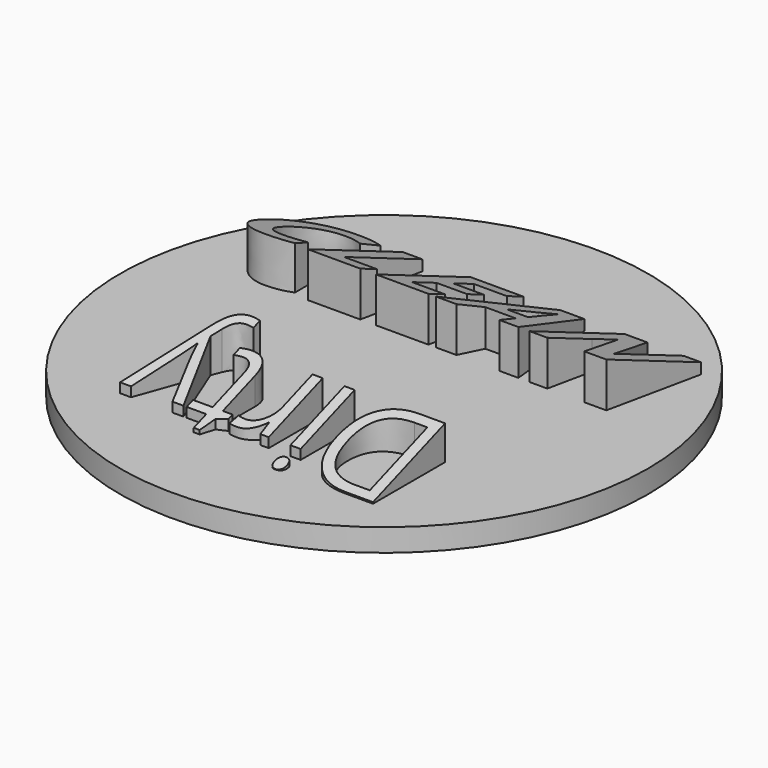
from build123d import *

# Parameters (mm, degrees)
F0_R           = 35
F1_DEPTH       = 3
F2_TEXT_SIZE   = 17.4245682355
F2_TEXT_SIZE_2 = 16.7269261761
F3_DEPTH       = 6
F5_DEPTH       = 35.001
F5_DEPTH_BACK  = 35.001
F6_R           = 4.2
F7_DEPTH       = 2


# Not quite as in the source:
# - Text() gives the source's letters only with a copy of the font that has no kerning and outlines rounded to 1/6400 em; it was checked with that copy


with BuildPart() as f1:
    # F0 (on Top) → F1 (new body)
    with BuildSketch(Plane.XY):
        Circle(F0_R)
    extrude(amount=F1_DEPTH)

    # F6 (on face) → F7 (cut)
    with BuildSketch(Plane(origin=(0, 0, 0), x_dir=(1, 0, 0), z_dir=(0, 0, -1))):
        Circle(F6_R)
    extrude(amount=-F7_DEPTH, mode=Mode.SUBTRACT)


with BuildPart() as f3:
    # F2 (on face) → F3 (new body)
    with BuildSketch(Plane.XY.offset(3)):
        with Locations((-27.2231652792, 7.5)):
            Text('CLEAN', F2_TEXT_SIZE, font='Open Sans', font_style=FontStyle.BOLDITALIC, text_align=(TextAlign.LEFT, TextAlign.BOTTOM))
        with Locations(Location((19.3287472711, -12), (0, 0, 180))):
            Text('Dirty', F2_TEXT_SIZE_2, font='Open Sans', text_align=(TextAlign.LEFT, TextAlign.BOTTOM))
    extrude(amount=F3_DEPTH)

    # F4 (on Right) → F5 (cut, two sides)
    with BuildSketch(Plane.YZ) as f5_sk:
        Polygon((20.255268745, 9), (7.3284769064, 9), (20.255268745, 4.2950325462), align=None)
        Polygon((-24.31585488, 3.0543481045), (-7.9803105533, 9), (-24.31585488, 9), align=None)
    extrude(amount=-F5_DEPTH, mode=Mode.SUBTRACT)
    extrude(f5_sk.sketch, amount=F5_DEPTH_BACK, mode=Mode.SUBTRACT)


solid = Compound([f1.part, f3.part])
